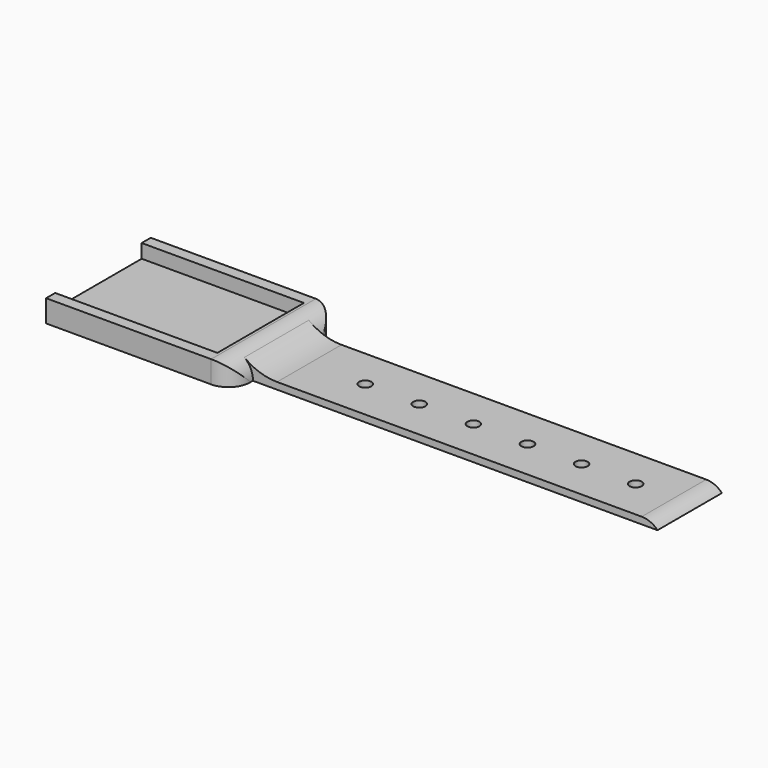
from build123d import *

# Parameters (mm, degrees)
F0_W         = 95.0192604214
F0_H         = 18.9093053341
F1_DEPTH     = 1.6002
F2_R         = 1.4351
F3_DEPTH     = 25.4
F4_R         = 1.397
F5_DEPTH     = 2.54
F6_W         = 48.927821219
F6_H         = 30.7276230305
F7_DEPTH     = 3.6195
F8_T1_DEPTH  = 30.6197
F8_T6_DEPTH  = 56.1276230305
F8_T12_DEPTH = 56.1276230305
F8_T18_DEPTH = 56.1276230305
F8_T25_DEPTH = 56.1276230305
F8_T31_DEPTH = 56.1276230305
F8_T37_DEPTH = 56.1276230305
F8_T43_DEPTH = 56.1276230305
F8_T49_DEPTH = 56.1276230305
F8_T56_DEPTH = 56.1276230305
F8_T62_DEPTH = 56.1276230305
F9_T1_DEPTH  = 37.4142992276
F10_R        = 12.7
F12_R        = 33.1286185238
F13_DEPTH    = 102.87
F14_W        = 25.4
F14_H        = 4.064
F15_DEPTH    = 38.1


# Not quite as in the source:
# - a fillet or chamfer that OpenCascade refuses, or shapes differently, is made with other operations: its cross-section is extruded or revolved along the edge and cut away or added


with BuildPart() as f1:
    # F0 (on Top) → F1 (new body)
    with BuildSketch(Plane.XY):
        Polygon((-24.4639106095, -15.3638115153), (24.4639106095, -15.3638115153), (24.4639106095, -9.454652667), (24.4639106095, 9.454652667), (24.4639106095, 15.3638115153), (-24.4639106095, 15.3638115153), (-24.4639106095, 9.454652667), (-24.4639106095, -9.454652667), align=None)
        with Locations((71.9735408202, 0)):
            Rectangle(F0_W, F0_H)
        with Locations((-71.9735408202, 0)):
            Rectangle(F0_W, F0_H)
    extrude(amount=F1_DEPTH)

    # F2 (on face) → F3 (cut)
    with BuildSketch(Plane.XY.offset(1.6002)):
        with Locations((106.7831710309, 0)):
            Circle(F2_R)
        with Locations((94.0831710309, 0)):
            Circle(F2_R)
        with Locations((81.3831710309, 0)):
            Circle(F2_R)
        with Locations((68.6831710309, 0)):
            Circle(F2_R)
        with Locations((55.9831710309, 0)):
            Circle(F2_R)
        with Locations((43.2831710309, 0)):
            Circle(F2_R)
    extrude(amount=-F3_DEPTH, mode=Mode.SUBTRACT)

    # F4 (on face) → F5 (join)
    with BuildSketch(Plane.XY.offset(1.6002)):
        with Locations((-106.7719441229, 0)):
            Circle(F4_R)
        with Locations((-94.0719441229, 0)):
            Circle(F4_R)
        with Locations((-81.3719441229, 0)):
            Circle(F4_R)
        with Locations((-68.6719441229, 0)):
            Circle(F4_R)
        with Locations((-55.9719441229, 0)):
            Circle(F4_R)
        with Locations((-43.2719441229, 0)):
            Circle(F4_R)
    extrude(amount=F5_DEPTH)

    # F6 (on face) → F7 (join)
    with BuildSketch(Plane.XY.offset(1.6002)):
        Rectangle(F6_W, F6_H)
    extrude(amount=F7_DEPTH)

    # F8: fillet of radius 5.08 on 6 edges, made by hand

    # F8_s2 → F8_t1 (cut)
    with BuildSketch(Plane.XY.offset(-12.7)):
        with BuildLine():
            ThreePointArc((-19.3839106095, 15.3638115153), (-22.9760130579, 13.8759139637), (-24.4639106095, 10.2838115153))
            Line((-24.4639106095, 10.2838115153), (-24.4639106095, 15.3638115153))
            Line((-24.4639106095, 15.3638115153), (-19.3839106095, 15.3638115153))
        make_face()
        with BuildLine():
            ThreePointArc((-19.3839106095, -15.3638115153), (-22.9760130579, -13.8759139637), (-24.4639106095, -10.2838115153))
            Line((-24.4639106095, -10.2838115153), (-24.4639106095, -15.3638115153))
            Line((-24.4639106095, -15.3638115153), (-19.3839106095, -15.3638115153))
        make_face()
        with BuildLine():
            ThreePointArc((19.3839106095, -15.3638115153), (22.9760130579, -13.8759139637), (24.4639106095, -10.2838115153))
            Line((24.4639106095, -10.2838115153), (24.4639106095, -15.3638115153))
            Line((24.4639106095, -15.3638115153), (19.3839106095, -15.3638115153))
        make_face()
        with BuildLine():
            ThreePointArc((19.3839106095, 15.3638115153), (22.9760130579, 13.8759139637), (24.4639106095, 10.2838115153))
            Line((24.4639106095, 10.2838115153), (24.4639106095, 15.3638115153))
            Line((24.4639106095, 15.3638115153), (19.3839106095, 15.3638115153))
        make_face()
    extrude(amount=F8_T1_DEPTH, mode=Mode.SUBTRACT)


with BuildPart() as f8_tool4:
    # F8_s5 → F8_t6 (new body)
    with BuildSketch(Plane.XZ.offset(28.0638115153)):
        with BuildLine():
            ThreePointArc((24.4639106095, 0.1397), (22.9760130579, 3.7318024484), (19.3839106095, 5.2197))
            Line((19.3839106095, 5.2197), (24.4639106095, 5.2197))
            Line((24.4639106095, 5.2197), (24.4639106095, 0.1397))
        make_face()
    extrude(amount=-F8_T6_DEPTH)

    split(bisect_by=Plane.XY.offset(1.6002), keep=Keep.BOTTOM)

    split(bisect_by=Plane.XZ.offset(9.454652667), keep=Keep.TOP)


with BuildPart() as f1_1:
    add(f1.part)

    # F8_t3: cut F8_tool4
    add(f8_tool4.part, mode=Mode.SUBTRACT)


with BuildPart() as f8_tool10:
    # F8_s11 → F8_t12 (new body)
    with BuildSketch(Plane.XZ.offset(28.0638115153)):
        with BuildLine():
            ThreePointArc((24.4639106095, 0.1397), (22.9760130579, 3.7318024484), (19.3839106095, 5.2197))
            Line((19.3839106095, 5.2197), (24.4639106095, 5.2197))
            Line((24.4639106095, 5.2197), (24.4639106095, 0.1397))
        make_face()
    extrude(amount=-F8_T12_DEPTH)

    split(bisect_by=Plane.XY.offset(1.6002), keep=Keep.TOP)

    split(bisect_by=Plane.XZ.offset(9.454652667), keep=Keep.TOP)


with BuildPart() as f1_2:
    add(f1_1.part)

    # F8_t9: cut F8_tool10
    add(f8_tool10.part, mode=Mode.SUBTRACT)


with BuildPart() as f8_tool16:
    # F8_s17 → F8_t18 (new body)
    with BuildSketch(Plane.XZ.offset(28.0638115153)):
        with BuildLine():
            ThreePointArc((24.4639106095, 0.1397), (22.9760130579, 3.7318024484), (19.3839106095, 5.2197))
            Line((19.3839106095, 5.2197), (24.4639106095, 5.2197))
            Line((24.4639106095, 5.2197), (24.4639106095, 0.1397))
        make_face()
    extrude(amount=-F8_T18_DEPTH)

    split(bisect_by=Plane.XY.offset(1.6002), keep=Keep.TOP)

    split(bisect_by=Plane.XZ.offset(-9.454652667), keep=Keep.TOP)

    split(bisect_by=Plane.XZ.offset(9.454652667), keep=Keep.BOTTOM)


with BuildPart() as f1_3:
    add(f1_2.part)

    # F8_t15: cut F8_tool16
    add(f8_tool16.part, mode=Mode.SUBTRACT)


with BuildPart() as f8_tool23:
    # F8_s24 → F8_t25 (new body)
    with BuildSketch(Plane.XZ.offset(28.0638115153)):
        with BuildLine():
            ThreePointArc((24.4639106095, 0.1397), (22.9760130579, 3.7318024484), (19.3839106095, 5.2197))
            Line((19.3839106095, 5.2197), (24.4639106095, 5.2197))
            Line((24.4639106095, 5.2197), (24.4639106095, 0.1397))
        make_face()
    extrude(amount=-F8_T25_DEPTH)

    split(bisect_by=Plane.XY.offset(1.6002), keep=Keep.BOTTOM)

    split(bisect_by=Plane.XZ.offset(-9.454652667), keep=Keep.BOTTOM)


with BuildPart() as f1_4:
    add(f1_3.part)

    # F8_t22: cut F8_tool23
    add(f8_tool23.part, mode=Mode.SUBTRACT)


with BuildPart() as f8_tool29:
    # F8_s30 → F8_t31 (new body)
    with BuildSketch(Plane.XZ.offset(28.0638115153)):
        with BuildLine():
            ThreePointArc((24.4639106095, 0.1397), (22.9760130579, 3.7318024484), (19.3839106095, 5.2197))
            Line((19.3839106095, 5.2197), (24.4639106095, 5.2197))
            Line((24.4639106095, 5.2197), (24.4639106095, 0.1397))
        make_face()
    extrude(amount=-F8_T31_DEPTH)

    split(bisect_by=Plane.XY.offset(1.6002), keep=Keep.TOP)

    split(bisect_by=Plane.XZ.offset(-9.454652667), keep=Keep.BOTTOM)


with BuildPart() as f1_5:
    add(f1_4.part)

    # F8_t28: cut F8_tool29
    add(f8_tool29.part, mode=Mode.SUBTRACT)


with BuildPart() as f8_tool35:
    # F8_s36 → F8_t37 (new body)
    with BuildSketch(Plane.XZ.offset(-28.0638115153)):
        with BuildLine():
            ThreePointArc((-19.3839106095, 5.2197), (-22.9760130579, 3.7318024484), (-24.4639106095, 0.1397))
            Line((-24.4639106095, 0.1397), (-24.4639106095, 5.2197))
            Line((-24.4639106095, 5.2197), (-19.3839106095, 5.2197))
        make_face()
    extrude(amount=F8_T37_DEPTH)

    split(bisect_by=Plane.XZ.offset(-9.454652667), keep=Keep.BOTTOM)

    split(bisect_by=Plane.XY.offset(1.6002), keep=Keep.TOP)


with BuildPart() as f1_6:
    add(f1_5.part)

    # F8_t34: cut F8_tool35
    add(f8_tool35.part, mode=Mode.SUBTRACT)


with BuildPart() as f8_tool41:
    # F8_s42 → F8_t43 (new body)
    with BuildSketch(Plane.XZ.offset(-28.0638115153)):
        with BuildLine():
            ThreePointArc((-19.3839106095, 5.2197), (-22.9760130579, 3.7318024484), (-24.4639106095, 0.1397))
            Line((-24.4639106095, 0.1397), (-24.4639106095, 5.2197))
            Line((-24.4639106095, 5.2197), (-19.3839106095, 5.2197))
        make_face()
    extrude(amount=F8_T43_DEPTH)

    split(bisect_by=Plane.XZ.offset(-9.454652667), keep=Keep.BOTTOM)

    split(bisect_by=Plane.XY.offset(1.6002), keep=Keep.BOTTOM)


with BuildPart() as f1_7:
    add(f1_6.part)

    # F8_t40: cut F8_tool41
    add(f8_tool41.part, mode=Mode.SUBTRACT)


with BuildPart() as f8_tool47:
    # F8_s48 → F8_t49 (new body)
    with BuildSketch(Plane.XZ.offset(-28.0638115153)):
        with BuildLine():
            ThreePointArc((-19.3839106095, 5.2197), (-22.9760130579, 3.7318024484), (-24.4639106095, 0.1397))
            Line((-24.4639106095, 0.1397), (-24.4639106095, 5.2197))
            Line((-24.4639106095, 5.2197), (-19.3839106095, 5.2197))
        make_face()
    extrude(amount=F8_T49_DEPTH)

    split(bisect_by=Plane.XZ.offset(-9.454652667), keep=Keep.TOP)

    split(bisect_by=Plane.XY.offset(1.6002), keep=Keep.TOP)

    split(bisect_by=Plane.XZ.offset(9.454652667), keep=Keep.BOTTOM)


with BuildPart() as f1_8:
    add(f1_7.part)

    # F8_t46: cut F8_tool47
    add(f8_tool47.part, mode=Mode.SUBTRACT)


with BuildPart() as f8_tool54:
    # F8_s55 → F8_t56 (new body)
    with BuildSketch(Plane.XZ.offset(-28.0638115153)):
        with BuildLine():
            ThreePointArc((-19.3839106095, 5.2197), (-22.9760130579, 3.7318024484), (-24.4639106095, 0.1397))
            Line((-24.4639106095, 0.1397), (-24.4639106095, 5.2197))
            Line((-24.4639106095, 5.2197), (-19.3839106095, 5.2197))
        make_face()
    extrude(amount=F8_T56_DEPTH)

    split(bisect_by=Plane.XY.offset(1.6002), keep=Keep.TOP)

    split(bisect_by=Plane.XZ.offset(9.454652667), keep=Keep.TOP)


with BuildPart() as f1_9:
    add(f1_8.part)

    # F8_t53: cut F8_tool54
    add(f8_tool54.part, mode=Mode.SUBTRACT)


with BuildPart() as f8_tool60:
    # F8_s61 → F8_t62 (new body)
    with BuildSketch(Plane.XZ.offset(-28.0638115153)):
        with BuildLine():
            ThreePointArc((-19.3839106095, 5.2197), (-22.9760130579, 3.7318024484), (-24.4639106095, 0.1397))
            Line((-24.4639106095, 0.1397), (-24.4639106095, 5.2197))
            Line((-24.4639106095, 5.2197), (-19.3839106095, 5.2197))
        make_face()
    extrude(amount=F8_T62_DEPTH)

    split(bisect_by=Plane.XY.offset(1.6002), keep=Keep.BOTTOM)

    split(bisect_by=Plane.XZ.offset(9.454652667), keep=Keep.TOP)


with BuildPart() as f1_10:
    add(f1_9.part)

    # F8_t59: cut F8_tool60
    add(f8_tool60.part, mode=Mode.SUBTRACT)

    # F9: fillet of radius 5.08 on 2 edges, made by hand

    # F9_s2 → F9_t1 (cut)
    with BuildSketch(Plane.XZ.offset(-18.7071496138)):
        with BuildLine():
            ThreePointArc((115.7821722522, 1.6002), (117.7982347512, 1.1830201767), (119.4831710309, 0))
            Line((119.4831710309, 0), (119.4831710309, 1.6002))
            Line((119.4831710309, 1.6002), (115.7821722522, 1.6002))
        make_face()
        with BuildLine():
            ThreePointArc((-119.4831710309, 0), (-117.7982347512, 1.1830201767), (-115.7821722522, 1.6002))
            Line((-115.7821722522, 1.6002), (-119.4831710309, 1.6002))
            Line((-119.4831710309, 1.6002), (-119.4831710309, 0))
        make_face()
    extrude(amount=F9_T1_DEPTH, mode=Mode.SUBTRACT)

    # F10
    f10_edges = [f1_10.edges().sort_by_distance(p)[0] for p in [
        (24.249436, 0, 1.6002),
        (-24.249436, 0, 1.6002),
    ]]
    fillet(f10_edges, radius=F10_R)

    # F12 (on offset) → F13 (cut)
    with BuildSketch(Plane.YZ.offset(-19.3802)):
        Circle(F12_R)
    extrude(amount=-F13_DEPTH, mode=Mode.SUBTRACT)

    # F14 (on offset) → F15 (cut)
    with BuildSketch(Plane.YZ.offset(-19.3802)):
        with Locations((0, 4.0005)):
            Rectangle(F14_W, F14_H)
    extrude(amount=F15_DEPTH, mode=Mode.SUBTRACT)


solid = f1_10.part
